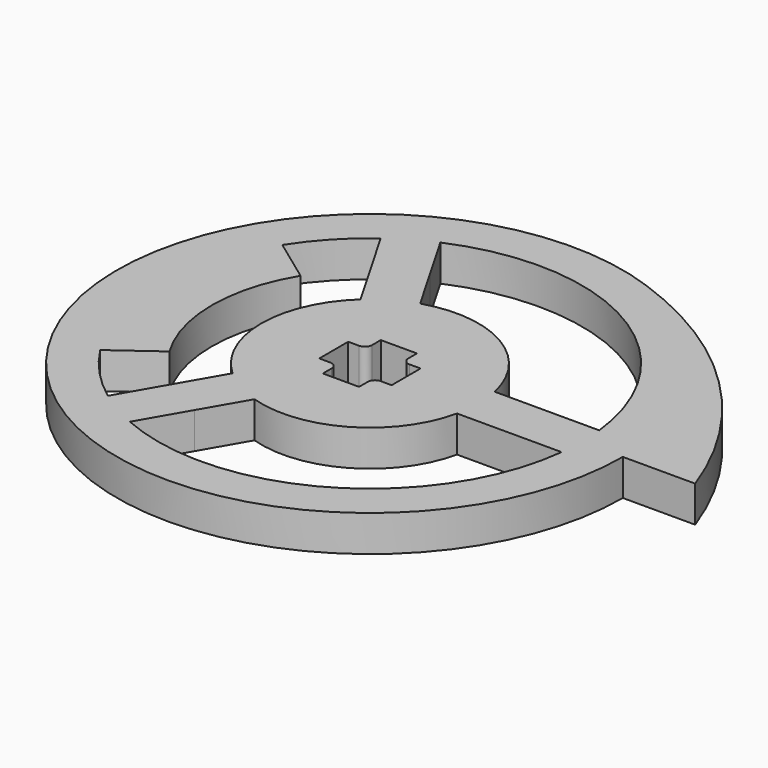
from build123d import *

# Parameters (mm, degrees)
F1_DEPTH = 6.35
F2_R     = 1.27


with BuildPart() as f1:
    # F0 (on Top) → F1 (new body)
    with BuildSketch(Plane.XY):
        with BuildLine():
            ThreePointArc((15.1071694838, 41.7235677075), (-36.3280432516, -25.4824634909), (44.3743470042, 0))
            ThreePointArc((44.3743470042, 0), (36.3280432516, 25.4824634909), (15.1071694838, 41.7235677075))
        make_face()
        with BuildLine():
            ThreePointArc((-14.8868357383, 34.0501787057), (18.5811231374, 32.1834493357), (36.9317376317, 4.1327114215))
            ThreePointArc((36.9317376317, 4.1327114215), (37.1045743636, 2.0695674625), (37.1622462748, 0))
            ThreePointArc((37.1622462748, 0), (37.1045743636, -2.0695674625), (36.9317376317, -4.1327114215))
            ThreePointArc((36.9317376317, -4.1327114215), (18.5811231374, -32.1834493357), (-14.8868357383, -34.0501787057))
            ThreePointArc((-14.8868357383, -34.0501787057), (-18.5811231374, -32.1834493357), (-22.0449018934, -29.9174672842))
            ThreePointArc((-22.0449018934, -29.9174672842), (-27.1515852785, -25.3736864695), (-31.3396552702, -19.9714435065))
            ThreePointArc((-31.3396552702, -19.9714435065), (-37.1622462748, 0), (-31.3396552702, 19.9714435065))
            ThreePointArc((-31.3396552702, 19.9714435065), (-27.1515852785, 25.3736864695), (-22.0449018934, 29.9174672842))
            ThreePointArc((-22.0449018934, 29.9174672842), (-18.5811231374, 32.1834493357), (-14.8868357383, 34.0501787057))
        make_face(mode=Mode.SUBTRACT)
        with BuildLine():
            ThreePointArc((15.1071694838, 41.7235677075), (36.3280432516, 25.4824634909), (44.3743470042, 0))
            Line((44.3743470042, 0), (57.0743470042, 0))
            ThreePointArc((57.0743470042, 0), (40.7796227308, 25.5780250359), (15.1071694838, 41.7235677075))
        make_face()
        with BuildLine():
            ThreePointArc((-9.525, 16.4977839421), (-7.6678534057, 17.4386502961), (-5.7191279813, 18.1712430817))
            Line((-5.7191279813, 18.1712430817), (-10.11946405, 25.792848723))
            ThreePointArc((-10.11946405, 25.792848723), (-13.8534706654, 23.9949150536), (-17.2775302051, 21.6601373015))
            Line((-17.2775302051, 21.6601373015), (-12.8771941364, 14.0385316602))
            ThreePointArc((-12.8771941364, 14.0385316602), (-11.2683874613, 15.3598809898), (-9.525, 16.4977839421))
        make_face()
        with BuildLine():
            ThreePointArc((-17.2775302051, 21.6601373015), (-13.8534706654, 23.9949150536), (-10.11946405, 25.792848723))
            Line((-10.11946405, 25.792848723), (-14.8868357383, 34.0501787057))
            ThreePointArc((-14.8868357383, 34.0501787057), (-18.5811231374, 32.1834493357), (-22.0449018934, 29.9174672842))
            Line((-22.0449018934, 29.9174672842), (-17.2775302051, 21.6601373015))
        make_face()
        with BuildLine():
            Line((-10.11946405, -25.792848723), (-5.7191279813, -18.1712430817))
            ThreePointArc((-5.7191279813, -18.1712430817), (-7.6678534057, -17.4386502961), (-9.525, -16.4977839421))
            ThreePointArc((-9.525, -16.4977839421), (-11.2683874613, -15.3598809898), (-12.8771941364, -14.0385316602))
            Line((-12.8771941364, -14.0385316602), (-17.2775302051, -21.6601373015))
            ThreePointArc((-17.2775302051, -21.6601373015), (-13.8534706654, -23.9949150536), (-10.11946405, -25.792848723))
        make_face()
        with BuildLine():
            Line((-14.8868357383, -34.0501787057), (-10.11946405, -25.792848723))
            ThreePointArc((-10.11946405, -25.792848723), (-13.8534706654, -23.9949150536), (-17.2775302051, -21.6601373015))
            Line((-17.2775302051, -21.6601373015), (-22.0449018934, -29.9174672842))
            ThreePointArc((-22.0449018934, -29.9174672842), (-18.5811231374, -32.1834493357), (-14.8868357383, -34.0501787057))
        make_face()
        with BuildLine():
            ThreePointArc((18.5963221177, 4.1327114215), (18.936240867, 2.0787693062), (19.05, 0))
            ThreePointArc((19.05, 0), (18.936240867, -2.0787693062), (18.5963221177, -4.1327114215))
            Line((18.5963221177, -4.1327114215), (27.3969942551, -4.1327114215))
            ThreePointArc((27.3969942551, -4.1327114215), (27.6293459059, -2.0721589516), (27.7069413308, 0))
            ThreePointArc((27.7069413308, 0), (27.6293459059, 2.0721589516), (27.3969942551, 4.1327114215))
            Line((27.3969942551, 4.1327114215), (18.5963221177, 4.1327114215))
        make_face()
        with BuildLine():
            Line((36.9317376317, 4.1327114215), (27.3969942551, 4.1327114215))
            ThreePointArc((27.3969942551, 4.1327114215), (27.6293459059, 2.0721589516), (27.7069413308, 0))
            ThreePointArc((27.7069413308, 0), (27.6293459059, -2.0721589516), (27.3969942551, -4.1327114215))
            Line((27.3969942551, -4.1327114215), (36.9317376317, -4.1327114215))
            ThreePointArc((36.9317376317, -4.1327114215), (37.1045743636, -2.0695674625), (37.1622462748, 0))
            ThreePointArc((37.1622462748, 0), (37.1045743636, 2.0695674625), (36.9317376317, 4.1327114215))
        make_face()
        with BuildLine():
            ThreePointArc((18.5963221177, -4.1327114215), (18.936240867, -2.0787693062), (19.05, 0))
            ThreePointArc((19.05, 0), (18.936240867, 2.0787693062), (18.5963221177, 4.1327114215))
            ThreePointArc((18.5963221177, 4.1327114215), (9.525, 16.4977839421), (-5.7191279813, 18.1712430817))
            ThreePointArc((-5.7191279813, 18.1712430817), (-7.6678534057, 17.4386502961), (-9.525, 16.4977839421))
            ThreePointArc((-9.525, 16.4977839421), (-11.2683874613, 15.3598809898), (-12.8771941364, 14.0385316602))
            ThreePointArc((-12.8771941364, 14.0385316602), (-19.05, 0), (-12.8771941364, -14.0385316602))
            ThreePointArc((-12.8771941364, -14.0385316602), (-11.2683874613, -15.3598809898), (-9.525, -16.4977839421))
            ThreePointArc((-9.525, -16.4977839421), (-7.6678534057, -17.4386502961), (-5.7191279813, -18.1712430817))
            ThreePointArc((-5.7191279813, -18.1712430817), (9.525, -16.4977839421), (18.5963221177, -4.1327114215))
        make_face()
        Polygon((-3.175, 6.35), (3.175, 6.35), (3.175, 3.175), (6.35, 3.175), (6.35, -3.175), (3.175, -3.175), (3.175, -6.35), (-3.175, -6.35), (-3.175, -3.175), (-6.35, -3.175), (-6.35, 3.175), (-3.175, 3.175), align=None, mode=Mode.SUBTRACT)
        with BuildLine():
            ThreePointArc((-23.6801005032, -14.3849726474), (-27.7069413308, 0), (-23.6801005032, 14.3849726474))
            Line((-23.6801005032, 14.3849726474), (-31.3396552702, 19.9714435065))
            ThreePointArc((-31.3396552702, 19.9714435065), (-37.1622462748, 0), (-31.3396552702, -19.9714435065))
            Line((-31.3396552702, -19.9714435065), (-23.6801005032, -14.3849726474))
        make_face()
    extrude(amount=F1_DEPTH)

    # F2
    f2_edges = [f1.edges().sort_by_distance(p)[0] for p in [
        (-3.175, 3.175, 3.175),
        (-3.175, -3.175, 3.175),
        (3.175, -3.175, 3.175),
        (3.175, 3.175, 3.175),
    ]]
    fillet(f2_edges, radius=F2_R)


solid = f1.part
